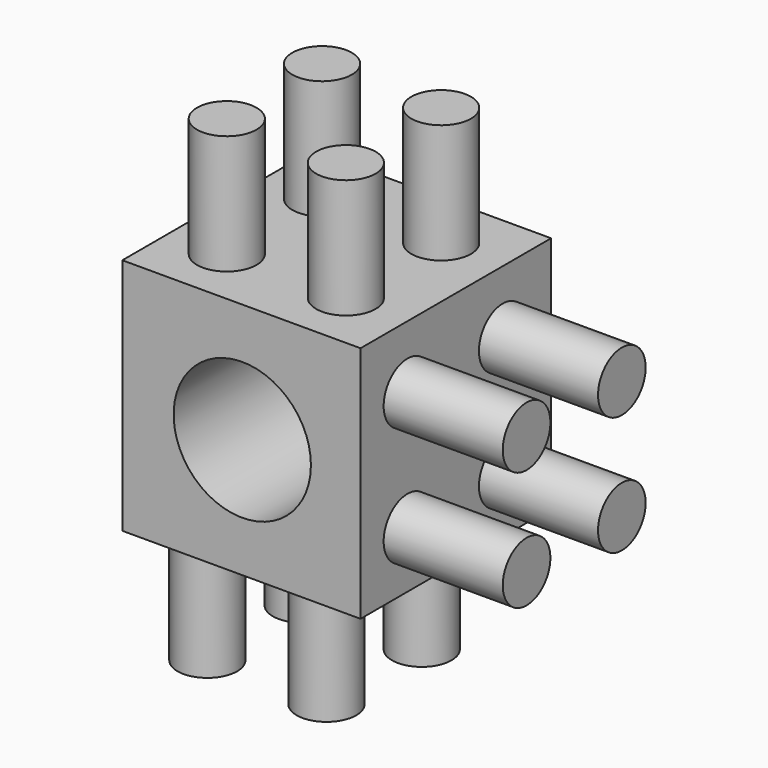
from build123d import *

# Parameters (mm, degrees)
F0_W     = 50.8
F0_H     = 50.8
F0_R     = 14.6377609255
F1_DEPTH = 50.8
F2_R     = 6.35
F3_DEPTH = 25.4
F4_R     = 6.35
F5_DEPTH = 25.4
F6_R     = 6.35
F7_DEPTH = 25.4


# Not quite as in the source:
# - the program builds the solid bodies; features that only make, move or delete a surface that nothing else refers to are left out


with BuildPart() as f1:
    # F0 (on Front) → F1 (new body)
    with BuildSketch(Plane.XZ):
        with Locations((25.4, -25.4)):
            Rectangle(F0_W, F0_H)
        with Locations((25.5802143365, -25.4)):
            Circle(F0_R, mode=Mode.SUBTRACT)
    extrude(amount=F1_DEPTH)


with BuildPart() as f3:
    # F2 (on Top) → F3 (new body)
    with BuildSketch(Plane.XY):
        with Locations((37.5657010168, -12.7627896145)):
            Circle(F2_R)
    extrude(amount=F3_DEPTH)


with BuildPart() as f3b:
    # F2 (on Top) → F3, piece 2 (new body)
    with BuildSketch(Plane.XY):
        with Locations((37.5657010168, -38.1627896145)):
            Circle(F2_R)
    extrude(amount=F3_DEPTH)


with BuildPart() as f3c:
    # F2 (on Top) → F3, piece 3 (new body)
    with BuildSketch(Plane.XY):
        with Locations((12.1657010168, -38.1627896145)):
            Circle(F2_R)
    extrude(amount=F3_DEPTH)


with BuildPart() as f3d:
    # F2 (on Top) → F3, piece 4 (new body)
    with BuildSketch(Plane.XY):
        with Locations((12.1657010168, -12.7627896145)):
            Circle(F2_R)
    extrude(amount=F3_DEPTH)


with BuildPart() as f5:
    # F4 (on face) → F5 (new body)
    with BuildSketch(Plane.YZ.offset(50.8)):
        with Locations((-12.8883697748, -38.7598782122)):
            Circle(F4_R)
    extrude(amount=F5_DEPTH)


with BuildPart() as f5b:
    # F4 (on face) → F5, piece 2 (new body)
    with BuildSketch(Plane.YZ.offset(50.8)):
        with Locations((-12.8883697748, -13.3598782122)):
            Circle(F4_R)
    extrude(amount=F5_DEPTH)


with BuildPart() as f5c:
    # F4 (on face) → F5, piece 3 (new body)
    with BuildSketch(Plane.YZ.offset(50.8)):
        with Locations((-38.2883697748, -13.3598782122)):
            Circle(F4_R)
    extrude(amount=F5_DEPTH)


with BuildPart() as f5d:
    # F4 (on face) → F5, piece 4 (new body)
    with BuildSketch(Plane.YZ.offset(50.8)):
        with Locations((-38.2883697748, -38.7598782122)):
            Circle(F4_R)
    extrude(amount=F5_DEPTH)


with BuildPart() as f7:
    # F6 (on face) → F7 (new body)
    with BuildSketch(Plane(origin=(0, 0, -50.8), x_dir=(1, 0, 0), z_dir=(0, 0, -1))):
        with Locations((9.7525073215, 40.323510766)):
            Circle(F6_R)
    extrude(amount=F7_DEPTH)


with BuildPart() as f7b:
    # F6 (on face) → F7, piece 2 (new body)
    with BuildSketch(Plane(origin=(0, 0, -50.8), x_dir=(1, 0, 0), z_dir=(0, 0, -1))):
        with Locations((35.1525073215, 14.923510766)):
            Circle(F6_R)
    extrude(amount=F7_DEPTH)


with BuildPart() as f7c:
    # F6 (on face) → F7, piece 3 (new body)
    with BuildSketch(Plane(origin=(0, 0, -50.8), x_dir=(1, 0, 0), z_dir=(0, 0, -1))):
        with Locations((9.7525073215, 14.923510766)):
            Circle(F6_R)
    extrude(amount=F7_DEPTH)


with BuildPart() as f7d:
    # F6 (on face) → F7, piece 4 (new body)
    with BuildSketch(Plane(origin=(0, 0, -50.8), x_dir=(1, 0, 0), z_dir=(0, 0, -1))):
        with Locations((35.1525073215, 40.323510766)):
            Circle(F6_R)
    extrude(amount=F7_DEPTH)


solid = Compound([f1.part, f3.part, f3b.part, f3c.part, f3d.part, f5.part, f5b.part, f5c.part, f5d.part, f7.part, f7b.part, f7c.part, f7d.part])
